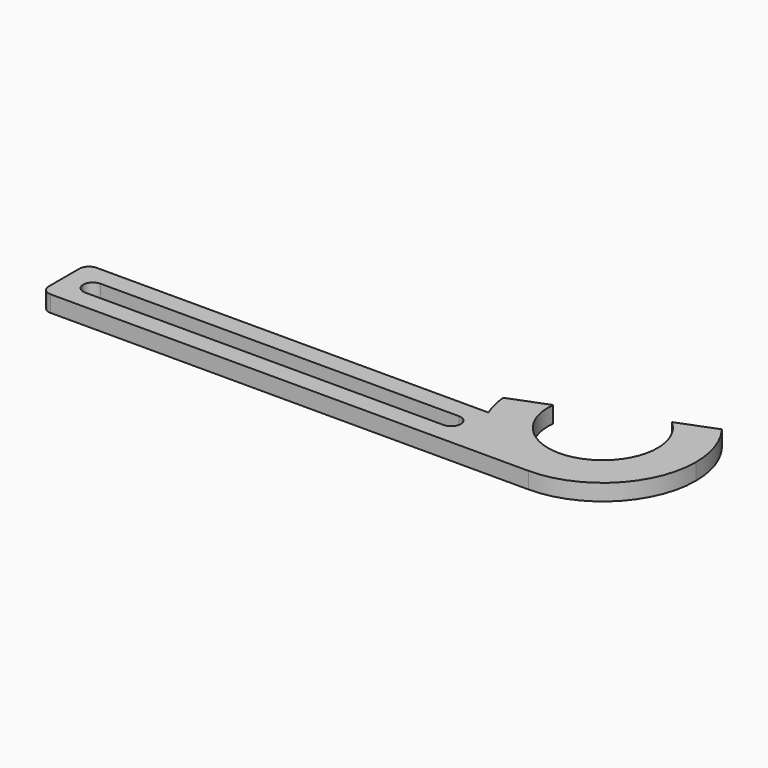
from build123d import *

# Parameters (mm, degrees)
F1_W     = 68.9904686213
F1_H     = 3.5
F2_DEPTH = 3
F3_R     = 1.74999


# Not quite as in the source:
# - a fillet or chamfer is up to 0.001 mm smaller than in the source, because OpenCascade refuses the exact size


with BuildPart() as f2:
    # F1 (on Top) → F2 (new body)
    with BuildSketch(Plane.XY):
        with BuildLine():
            Line((0, 10.5), (0, 0))
            Line((0, 0), (89.0564994759, 0))
            ThreePointArc((89.0564994759, 0), (79.609277662, 2.8667059749), (73.3482214035, 10.5))
            Line((73.3482214035, 10.5), (59.6541650593, 10.5))
            Line((59.6541650593, 10.5), (0, 10.5))
        make_face()
        with Locations((37.9952343106, 5.25)):
            Rectangle(F1_W, F1_H, mode=Mode.SUBTRACT)
        with BuildLine():
            ThreePointArc((73.3482214035, 10.5), (79.609277662, 2.8667059749), (89.0564994759, 0))
            ThreePointArc((89.0564994759, 0), (101.0773147561, 4.9791847198), (106.0564994759, 17))
            ThreePointArc((106.0564994759, 17), (105.1713324233, 22.414070472), (102.6080101728, 27.2643342614))
            Line((102.6080101728, 27.2643342614), (95.6259965732, 24.5393439959))
            ThreePointArc((95.6259965732, 24.5393439959), (98.158558885, 21.1415594301), (99.0564994759, 17))
            ThreePointArc((99.0564994759, 17), (88.5076755448, 7.0150717432), (79.1167410173, 18.0959935155))
            Line((79.1167410173, 18.0959935155), (72.1347274177, 15.37100325))
            ThreePointArc((72.1347274177, 15.37100325), (72.5606905825, 12.8904636571), (73.3482214035, 10.5))
        make_face()
    extrude(amount=F2_DEPTH)

    # F3 (radius 1.75 in the source; OpenCascade refuses exactly that, so slightly less here)
    f3_edges = [f2.edges().sort_by_distance(p)[0] for p in [
        (3.5, 7, 1.5),
        (3.5, 3.5, 1.5),
        (0, 10.5, 1.5),
        (0, 0, 1.5),
        (72.490469, 7, 1.5),
        (72.490469, 3.5, 1.5),
    ]]
    fillet(f3_edges, radius=F3_R)


solid = f2.part
